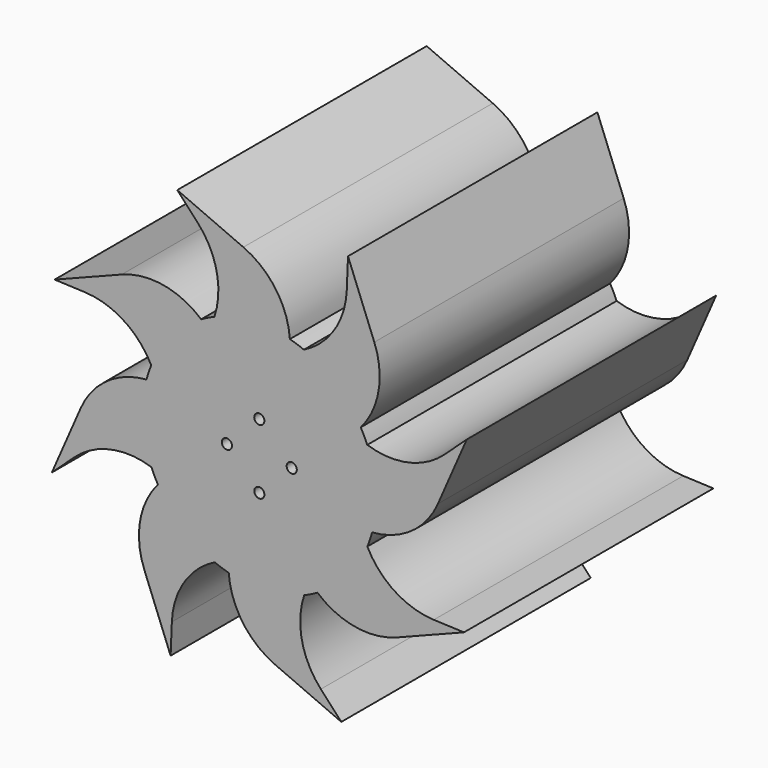
from build123d import *

# Parameters (mm, degrees)
F1_DEPTH    = 101.6
F2_T1_DEPTH = 101.6
F2_T3_DEPTH = 213.9945264783
F3_R        = 1.651
F4_DEPTH    = 127
F5_R        = 3.81
F5_R_2      = 1.651
F6_DEPTH    = 98.425


# Not quite as in the source:
# - a fillet or chamfer that OpenCascade refuses, or shapes differently, is made with other operations: its cross-section is extruded or revolved along the edge and cut away or added


with BuildPart() as f1:
    # F0 (on Front) → F1 (new body)
    with BuildSketch(Plane.XZ):
        with BuildLine():
            ThreePointArc((36.7729649274, -9.9679010051), (37.7667841081, -5.0279238392), (38.1, 0))
            ThreePointArc((38.1, 0), (37.363123518, 7.4570101903), (35.1809973239, 14.6255744261))
            ThreePointArc((35.1809973239, 14.6255744261), (34.1844683928, 16.823558503), (33.0507832594, 18.9540424696))
            ThreePointArc((33.0507832594, 18.9540424696), (25.1442335653, 28.6247710631), (14.5348789212, 35.2185646321))
            ThreePointArc((14.5348789212, 35.2185646321), (12.2760171106, 36.068121713), (9.9679010051, 36.7729649274))
            ThreePointArc((9.9679010051, 36.7729649274), (-2.4611116668, 38.0204277904), (-14.6255744261, 35.1809973239))
            ThreePointArc((-14.6255744261, 35.1809973239), (-16.823558503, 34.1844683928), (-18.9540424696, 33.0507832594))
            ThreePointArc((-18.9540424696, 33.0507832594), (-28.6247710631, 25.1442335653), (-35.2185646321, 14.5348789212))
            ThreePointArc((-35.2185646321, 14.5348789212), (-36.068121713, 12.2760171106), (-36.7729649274, 9.9679010051))
            ThreePointArc((-36.7729649274, 9.9679010051), (-38.0204277904, -2.4611116668), (-35.1809973239, -14.6255744261))
            ThreePointArc((-35.1809973239, -14.6255744261), (-34.1844683928, -16.823558503), (-33.0507832594, -18.9540424696))
            ThreePointArc((-33.0507832594, -18.9540424696), (-25.1442335653, -28.6247710631), (-14.5348789212, -35.2185646321))
            ThreePointArc((-14.5348789212, -35.2185646321), (-12.2760171106, -36.068121713), (-9.9679010051, -36.7729649274))
            ThreePointArc((-9.9679010051, -36.7729649274), (2.4611116668, -38.0204277904), (14.6255744261, -35.1809973239))
            ThreePointArc((14.6255744261, -35.1809973239), (16.823558503, -34.1844683928), (18.9540424696, -33.0507832594))
            ThreePointArc((18.9540424696, -33.0507832594), (28.6247710631, -25.1442335653), (35.2185646321, -14.5348789212))
            ThreePointArc((35.2185646321, -14.5348789212), (36.068121713, -12.2760171106), (36.7729649274, -9.9679010051))
        make_face()
        with BuildLine():
            ThreePointArc((-35.2185646321, 14.5348789212), (-28.6247710631, 25.1442335653), (-18.9540424696, 33.0507832594))
            Line((-18.9540424696, 33.0507832594), (-23.9079516621, 45.688308647))
            Line((-23.9079516621, 45.688308647), (-66.712088778, 28.9090894698))
            Line((-66.712088778, 28.9090894698), (-41.705504873, 27.890755436))
            Line((-41.705504873, 27.890755436), (-35.2185646321, 14.5348789212))
        make_face()
        with BuildLine():
            ThreePointArc((-14.6255744261, 35.1809973239), (-2.4611116668, 38.0204277904), (9.9679010051, 36.7729649274))
            Line((9.9679010051, 36.7729649274), (15.4010381207, 49.2119876098))
            Line((15.4010381207, 49.2119876098), (-26.7307571601, 67.6143835641))
            Line((-26.7307571601, 67.6143835641), (-9.7685030073, 49.2119876098))
            Line((-9.7685030073, 49.2119876098), (-14.6255744261, 35.1809973239))
        make_face()
        with BuildLine():
            ThreePointArc((14.5348789212, 35.2185646321), (25.1442335653, 28.6247710631), (33.0507832594, 18.9540424696))
            Line((33.0507832594, 18.9540424696), (45.688308647, 23.9079516621))
            Line((45.688308647, 23.9079516621), (28.9090894698, 66.712088778))
            Line((28.9090894698, 66.712088778), (27.890755436, 41.705504873))
            Line((27.890755436, 41.705504873), (14.5348789212, 35.2185646321))
        make_face()
        with BuildLine():
            ThreePointArc((35.1809973239, 14.6255744261), (37.363123518, 7.4570101903), (38.1, 0))
            ThreePointArc((38.1, 0), (37.7667841081, -5.0279238392), (36.7729649274, -9.9679010051))
            Line((36.7729649274, -9.9679010051), (49.2119876098, -15.4010381207))
            Line((49.2119876098, -15.4010381207), (67.6143835641, 26.7307571601))
            Line((67.6143835641, 26.7307571601), (49.2119876098, 9.7685030073))
            Line((49.2119876098, 9.7685030073), (35.1809973239, 14.6255744261))
        make_face()
        with BuildLine():
            Line((41.705504873, -27.890755436), (35.2185646321, -14.5348789212))
            ThreePointArc((35.2185646321, -14.5348789212), (28.6247710631, -25.1442335653), (18.9540424696, -33.0507832594))
            Line((18.9540424696, -33.0507832594), (23.9079516621, -45.688308647))
            Line((23.9079516621, -45.688308647), (66.712088778, -28.9090894698))
            Line((66.712088778, -28.9090894698), (41.705504873, -27.890755436))
        make_face()
        with BuildLine():
            Line((9.7685030073, -49.2119876098), (14.6255744261, -35.1809973239))
            ThreePointArc((14.6255744261, -35.1809973239), (2.4611116668, -38.0204277904), (-9.9679010051, -36.7729649274))
            Line((-9.9679010051, -36.7729649274), (-15.4010381207, -49.2119876098))
            Line((-15.4010381207, -49.2119876098), (26.7307571601, -67.6143835641))
            Line((26.7307571601, -67.6143835641), (9.7685030073, -49.2119876098))
        make_face()
        with BuildLine():
            Line((-27.890755436, -41.705504873), (-14.5348789212, -35.2185646321))
            ThreePointArc((-14.5348789212, -35.2185646321), (-25.1442335653, -28.6247710631), (-33.0507832594, -18.9540424696))
            Line((-33.0507832594, -18.9540424696), (-45.688308647, -23.9079516621))
            Line((-45.688308647, -23.9079516621), (-28.9090894698, -66.712088778))
            Line((-28.9090894698, -66.712088778), (-27.890755436, -41.705504873))
        make_face()
        with BuildLine():
            ThreePointArc((-35.1809973239, -14.6255744261), (-38.0204277904, -2.4611116668), (-36.7729649274, 9.9679010051))
            Line((-36.7729649274, 9.9679010051), (-49.2119876098, 15.4010381207))
            Line((-49.2119876098, 15.4010381207), (-67.6143835641, -26.7307571601))
            Line((-67.6143835641, -26.7307571601), (-49.2119876098, -9.7685030073))
            Line((-49.2119876098, -9.7685030073), (-35.1809973239, -14.6255744261))
        make_face()
    extrude(amount=F1_DEPTH)

    # F2: fillet of radius 25.4 on 16 edges, made by hand

    # F2_s2 → F2_t1 (join)
    with BuildSketch(Plane.XZ):
        with BuildLine():
            ThreePointArc((-56.8805102577, 28.5087216686), (-44.1451035636, 24.4740120759), (-35.2185646321, 14.5348789212))
            Line((-35.2185646321, 14.5348789212), (-41.705504873, 27.890755436))
            Line((-41.705504873, 27.890755436), (-56.8805102577, 28.5087216686))
        make_face()
        with BuildLine():
            ThreePointArc((-60.3793049354, -20.0618841058), (-48.5210419877, -13.9095621843), (-35.1809973239, -14.6255744261))
            Line((-35.1809973239, -14.6255744261), (-49.2119876098, -9.7685030073))
            Line((-49.2119876098, -9.7685030073), (-60.3793049354, -20.0618841058))
        make_face()
        with BuildLine():
            ThreePointArc((-28.5087216686, -56.8805102577), (-24.4740120759, -44.1451035636), (-14.5348789212, -35.2185646321))
            Line((-14.5348789212, -35.2185646321), (-27.890755436, -41.705504873))
            Line((-27.890755436, -41.705504873), (-28.5087216686, -56.8805102577))
        make_face()
        with BuildLine():
            ThreePointArc((20.0618841058, -60.3793049354), (13.9095621843, -48.5210419877), (14.6255744261, -35.1809973239))
            Line((14.6255744261, -35.1809973239), (9.7685030073, -49.2119876098))
            Line((9.7685030073, -49.2119876098), (20.0618841058, -60.3793049354))
        make_face()
        with BuildLine():
            ThreePointArc((56.8805102577, -28.5087216686), (44.1451035636, -24.4740120759), (35.2185646321, -14.5348789212))
            Line((35.2185646321, -14.5348789212), (41.705504873, -27.890755436))
            Line((41.705504873, -27.890755436), (56.8805102577, -28.5087216686))
        make_face()
        with BuildLine():
            ThreePointArc((60.3793049354, 20.0618841058), (48.5210419877, 13.9095621843), (35.1809973239, 14.6255744261))
            Line((35.1809973239, 14.6255744261), (49.2119876098, 9.7685030073))
            Line((49.2119876098, 9.7685030073), (60.3793049354, 20.0618841058))
        make_face()
        with BuildLine():
            ThreePointArc((28.5087216686, 56.8805102577), (24.4740120759, 44.1451035636), (14.5348789212, 35.2185646321))
            Line((14.5348789212, 35.2185646321), (27.890755436, 41.705504873))
            Line((27.890755436, 41.705504873), (28.5087216686, 56.8805102577))
        make_face()
        with BuildLine():
            ThreePointArc((-20.0618841058, 60.3793049354), (-13.9095621843, 48.5210419877), (-14.6255744261, 35.1809973239))
            Line((-14.6255744261, 35.1809973239), (-9.7685030073, 49.2119876098))
            Line((-9.7685030073, 49.2119876098), (-20.0618841058, 60.3793049354))
        make_face()
    extrude(amount=F2_T1_DEPTH)

    # F2_s4 → F2_t3 (cut)
    with BuildSketch(Plane.XZ.offset(-56.1972632391)):
        with BuildLine():
            ThreePointArc((-36.7729649274, 9.9679010051), (-49.6032208566, 5.3697394136), (-58.2095345387, -5.1986058702))
            Line((-58.2095345387, -5.1986058702), (-49.2119876098, 15.4010381207))
            Line((-49.2119876098, 15.4010381207), (-36.7729649274, 9.9679010051))
        make_face()
        with BuildLine():
            ThreePointArc((-18.9540424696, 33.0507832594), (-31.2777946839, 38.8717529889), (-44.8363260656, 37.4843871385))
            Line((-44.8363260656, 37.4843871385), (-23.9079516621, 45.688308647))
            Line((-23.9079516621, 45.688308647), (-18.9540424696, 33.0507832594))
        make_face()
        with BuildLine():
            ThreePointArc((9.9679010051, 36.7729649274), (5.3697394136, 49.6032208566), (-5.1986058702, 58.2095345387))
            Line((-5.1986058702, 58.2095345387), (15.4010381207, 49.2119876098))
            Line((15.4010381207, 49.2119876098), (9.9679010051, 36.7729649274))
        make_face()
        with BuildLine():
            ThreePointArc((33.0507832594, 18.9540424696), (38.8717529889, 31.2777946839), (37.4843871385, 44.8363260656))
            Line((37.4843871385, 44.8363260656), (45.688308647, 23.9079516621))
            Line((45.688308647, 23.9079516621), (33.0507832594, 18.9540424696))
        make_face()
        with BuildLine():
            ThreePointArc((36.7729649274, -9.9679010051), (49.6032208566, -5.3697394136), (58.2095345387, 5.1986058702))
            Line((58.2095345387, 5.1986058702), (49.2119876098, -15.4010381207))
            Line((49.2119876098, -15.4010381207), (36.7729649274, -9.9679010051))
        make_face()
        with BuildLine():
            ThreePointArc((18.9540424696, -33.0507832594), (31.2777946839, -38.8717529889), (44.8363260656, -37.4843871385))
            Line((44.8363260656, -37.4843871385), (23.9079516621, -45.688308647))
            Line((23.9079516621, -45.688308647), (18.9540424696, -33.0507832594))
        make_face()
        with BuildLine():
            ThreePointArc((-9.9679010051, -36.7729649274), (-5.3697394136, -49.6032208566), (5.1986058702, -58.2095345387))
            Line((5.1986058702, -58.2095345387), (-15.4010381207, -49.2119876098))
            Line((-15.4010381207, -49.2119876098), (-9.9679010051, -36.7729649274))
        make_face()
        with BuildLine():
            ThreePointArc((-33.0507832594, -18.9540424696), (-38.8717529889, -31.2777946839), (-37.4843871385, -44.8363260656))
            Line((-37.4843871385, -44.8363260656), (-45.688308647, -23.9079516621))
            Line((-45.688308647, -23.9079516621), (-33.0507832594, -18.9540424696))
        make_face()
    extrude(amount=F2_T3_DEPTH, mode=Mode.SUBTRACT)

    # F3 (on face) → F4 (cut)
    with BuildSketch(Plane(origin=(0, 0, 0), x_dir=(-1, 0, 0), z_dir=(0, 1, 0))):
        with Locations((0, 10.5664)):
            Circle(F3_R)
        with Locations((-10.5664, 0)):
            Circle(F3_R)
        with Locations((10.5664, 0)):
            Circle(F3_R)
        with Locations((0, -10.5664)):
            Circle(F3_R)
    extrude(amount=-F4_DEPTH, mode=Mode.SUBTRACT)

    # F5 (on face) → F6 (cut)
    with BuildSketch(Plane(origin=(0, 0, 0), x_dir=(-1, 0, 0), z_dir=(0, 1, 0))):
        with Locations((0, 10.5664)):
            Circle(F5_R)
        with Locations((0, 10.5664)):
            Circle(F5_R_2, mode=Mode.SUBTRACT)
        with Locations((10.5664, 0)):
            Circle(F5_R)
        with Locations((10.5664, 0)):
            Circle(F5_R_2, mode=Mode.SUBTRACT)
        with Locations((0, -10.5664)):
            Circle(F5_R)
        with Locations((0, -10.5664)):
            Circle(F5_R_2, mode=Mode.SUBTRACT)
        with Locations((-10.5664, 0)):
            Circle(F5_R)
        with Locations((-10.5664, 0)):
            Circle(F5_R_2, mode=Mode.SUBTRACT)
    extrude(amount=-F6_DEPTH, mode=Mode.SUBTRACT)


solid = f1.part
